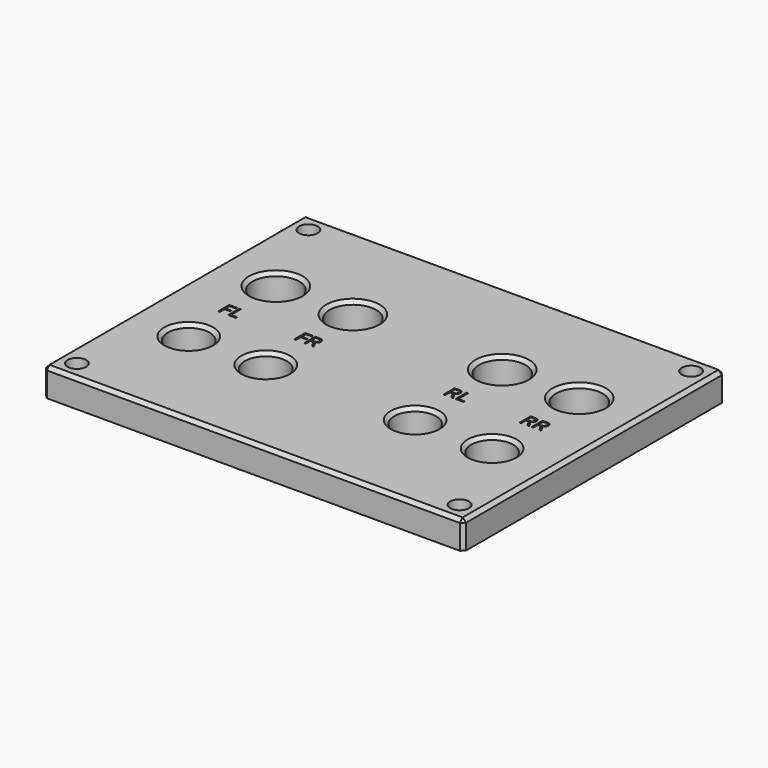
from build123d import *

# Parameters (mm, degrees)
F0_W           = 180
F0_H           = 140
F0_R           = 9
F0_R_2         = 10
F1_DEPTH       = 12
F2_SIZE        = 1.5
F3_SIZE        = 1.5
F4_D           = 4.2
F4_CBORE_D     = 8
F4_CBORE_DEPTH = 5
F5_TEXT_SIZE   = 8.3333333333
F6_DEPTH       = 1


# Not quite as in the source:
# - Text() gives the source's letters only with a copy of the font that has no kerning and outlines rounded to 1/6400 em; it was checked with that copy


with BuildPart() as f1:
    # F0 (on Top) → F1 (new body)
    with BuildSketch(Plane.XY):
        Rectangle(F0_W, F0_H)
        with Locations((-65, -23.3333333333)):
            Circle(F0_R, mode=Mode.SUBTRACT)
        with Locations((-32, -23.3333333333)):
            Circle(F0_R, mode=Mode.SUBTRACT)
        with Locations((32, -23.3333333333)):
            Circle(F0_R, mode=Mode.SUBTRACT)
        with Locations((65, -23.3333333333)):
            Circle(F0_R, mode=Mode.SUBTRACT)
        with Locations((-65, 23.3333333333)):
            Circle(F0_R_2, mode=Mode.SUBTRACT)
        with Locations((-32, 23.3333333333)):
            Circle(F0_R_2, mode=Mode.SUBTRACT)
        with Locations((32, 23.3333333333)):
            Circle(F0_R_2, mode=Mode.SUBTRACT)
        with Locations((65, 23.3333333333)):
            Circle(F0_R_2, mode=Mode.SUBTRACT)
    extrude(amount=-F1_DEPTH)

    # F2
    f2_edges = [f1.edges().sort_by_distance(p)[0] for p in [
        (-90, 70, -6),
        (90, 70, -6),
        (90, -70, -6),
        (-90, -70, -6),
        (0, 70, 0),
        (0, -70, 0),
        (-90, 0, 0),
        (90, 0, 0),
    ]]
    chamfer(f2_edges, length=F2_SIZE)

    # F3
    f3_edges = [f1.edges().sort_by_distance(p)[0] for p in [
        (-75, 23.333333, 0),
        (-42, 23.333333, 0),
        (22, 23.333333, 0),
        (55, 23.333333, 0),
        (-74, -23.333333, 0),
        (-41, -23.333333, 0),
        (23, -23.333333, 0),
        (56, -23.333333, 0),
    ]]
    chamfer(f3_edges, length=F3_SIZE)

    # F4 (through all)
    with Locations(Plane.XY):
        with Locations((82, 62), (82, -62), (-82, -62), (-82, 62)):
            CounterBoreHole(F4_D / 2, F4_CBORE_D / 2, F4_CBORE_DEPTH)

    # F5 (on Top) → F6 (cut)
    with BuildSketch(Plane.XY):
        with Locations((-69.4876302083, -3)):
            Text('FL', F5_TEXT_SIZE, font='Open Sans', text_align=(TextAlign.LEFT, TextAlign.BOTTOM))
        with Locations((-36.9251302083, -3)):
            Text('FR', F5_TEXT_SIZE, font='Open Sans', text_align=(TextAlign.LEFT, TextAlign.BOTTOM))
        with Locations((27.0872395833, -3)):
            Text('RL', F5_TEXT_SIZE, font='Open Sans', text_align=(TextAlign.LEFT, TextAlign.BOTTOM))
        with Locations((59.6497395833, -3)):
            Text('RR', F5_TEXT_SIZE, font='Open Sans', text_align=(TextAlign.LEFT, TextAlign.BOTTOM))
    extrude(amount=-F6_DEPTH, mode=Mode.SUBTRACT)


solid = f1.part
